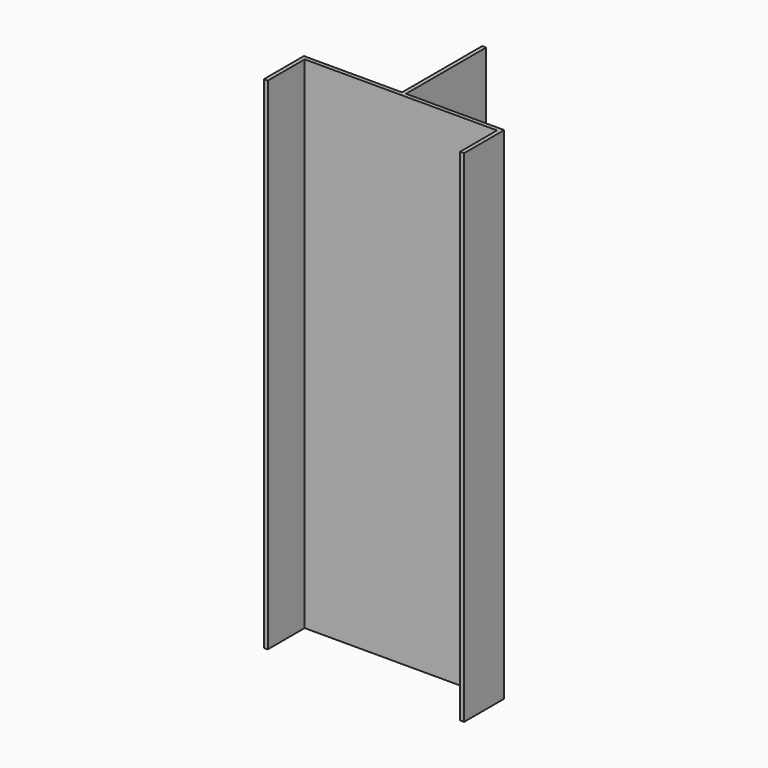
from build123d import *

# Parameters (mm, degrees)
F0_W     = 50.8
F0_H     = 12.7
F1_DEPTH = 127
F2_T     = -1
F3_W     = 50.8
F3_H     = 127
F4_DEPTH = 25.4
F5_W     = 24.9
F5_H     = 25.4
F6_DEPTH = 127


# Not quite as in the source:
# - a pattern or mirror of a feature is missing from the dataset's text; its kind, count and spacing are read off the source's solid


with BuildPart() as f1:
    # F0 (on Top) → F1 (new body)
    with BuildSketch(Plane.XY):
        Rectangle(F0_W, F0_H)
    extrude(amount=F1_DEPTH)

    # F2
    f2_openings = [f1.faces().sort_by_distance(p)[0] for p in [
        (0, 0, 127),
        (0, -6.35, 63.5),
        (0, 0, 0),
    ]]
    offset(amount=F2_T, openings=f2_openings)

    # F3 (on face) → F4 (join)
    with BuildSketch(Plane(origin=(0, 6.35, 0), x_dir=(-1, 0, 0), z_dir=(0, 1, 0))):
        with Locations((0, 63.5)):
            Rectangle(F3_W, F3_H)
    extrude(amount=F4_DEPTH)

    # F5 (on face) → F6 (cut)
    with BuildSketch(Plane.XY.offset(127)):
        with Locations((-12.95, 19.05)):
            Rectangle(F5_W, F5_H)
    f6 = extrude(amount=-F6_DEPTH, mode=Mode.SUBTRACT)

    # F6_copies: F6 across plane
    add(f6.mirror(Plane(origin=(0, 0, 0), x_dir=(0, 0, 1), z_dir=(1, 0, 0))), mode=Mode.SUBTRACT)


solid = f1.part
